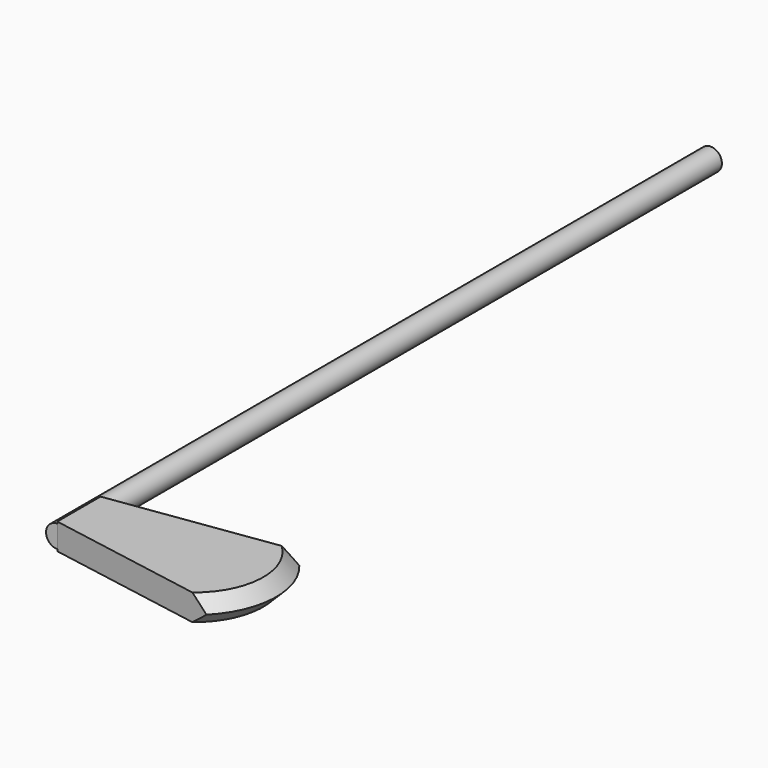
from build123d import *

# Parameters (mm, degrees)
F0_R          = 2.179542758
F1_DEPTH      = 158.64632
F3_DEPTH      = 2.54
F3_DEPTH_BACK = 2.54
F4_SIZE       = 2.53999


# Not quite as in the source:
# - a fillet or chamfer is up to 0.001 mm smaller than in the source, because OpenCascade refuses the exact size


with BuildPart() as f1:
    # F0 (on Front) → F1 (new body)
    with BuildSketch(Plane.XZ):
        Circle(F0_R)
    extrude(amount=-F1_DEPTH)


with BuildPart() as f3:
    # F2 (on Top) → F3 (new body, two sides)
    with BuildSketch(Plane.XY) as f3_sk:
        with BuildLine():
            Line((0, 10.5042038485), (0, 0))
            Line((0, 0), (33.7287560105, -5.9487139806))
            ThreePointArc((33.7287560105, -5.9487139806), (38.33498105, 4.5782306181), (34.6436500549, 15.4597721994))
            Line((34.6436500549, 15.4597721994), (0, 10.5042038485))
        make_face()
    extrude(amount=F3_DEPTH)
    extrude(f3_sk.sketch, amount=-F3_DEPTH_BACK)

    # F4 (size 2.54 in the source; OpenCascade refuses exactly that, so slightly less here)
    f4_edges = [f3.edges().sort_by_distance(p)[0] for p in [
        (38.334981, 4.578231, -2.54),
        (38.334981, 4.578231, 2.54),
    ]]
    chamfer(f4_edges, length=F4_SIZE)


solid = Compound([f1.part, f3.part])
